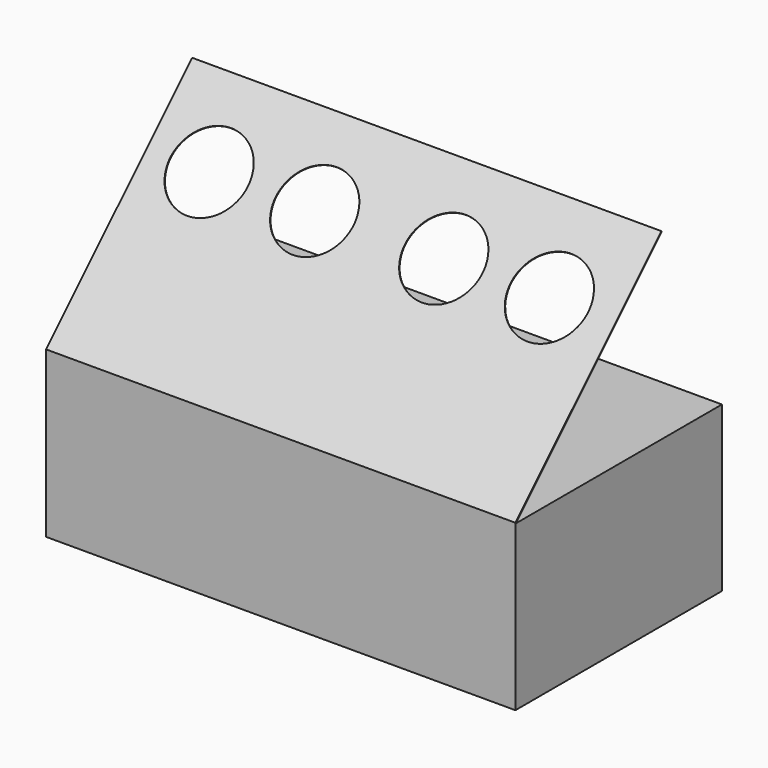
from build123d import *

# Parameters (mm, degrees)
F1_DEPTH = 127
F3_DEPTH = 0.4064


# Not quite as in the source:
# - the dataset's text gives a spline's control points without its knots; the knots are read off the source's solid


with BuildPart() as f1:
    # F0 (on Right) → F1 (new body, symmetric)
    with BuildSketch(Plane.YZ):
        Polygon((-139.7, 0), (0, 0), (0, 88.9), (-139.2936, 88.9), (-139.2936, 89.154), (-40.6298144724, 187.8177855276), (-40.9171826682, 188.1051537235), (-139.7, 89.3223363917), align=None)
    extrude(amount=F1_DEPTH, both=True)

    # F2 (on face) → F3 (cut, through all)
    with BuildSketch(Plane(origin=(0, -114.5111681959, 114.5111681959), x_dir=(1, 0, 0), z_dir=(0, -0.7071067812, 0.7071067812))):
        with BuildLine():
            add(Edge.make_bspline(
                [(-21.0882612312, 45.5766371575), (-17.1946190312, 49.4705841575), (-14.9277452312, 54.9434713575), (-14.9277452312, 60.4501405575), (-14.9277452312, 65.9570891575), (-17.1946190312, 71.4299763575), (-21.0882612312, 75.3236185575), (-24.9822590312, 79.2176163575), (-30.4551462312, 81.4845155575), (-35.9621202312, 81.4845155575)],
                knots=[5, 5, 5, 5, 6, 6, 6, 7, 7, 7, 8, 8, 8, 8], degree=3))
            add(Edge.make_bspline(
                [(-35.9621202312, 81.4845155575), (-41.4687640312, 81.4845155575), (-46.9416512312, 79.2176163575), (-50.8352934312, 75.3236185575)],
                knots=[0, 0, 0, 0, 1, 1, 1, 1], degree=3))
            add(Edge.make_bspline(
                [(-50.8352934312, 75.3236185575), (-54.7292912312, 71.4299763575), (-56.9964952312, 65.9570891575), (-56.9964952312, 60.4501405575), (-56.9964952312, 54.9434713575), (-54.7292912312, 49.4705841575), (-50.8352934312, 45.5766371575)],
                knots=[1, 1, 1, 1, 2, 2, 2, 3, 3, 3, 3], degree=3))
            add(Edge.make_bspline(
                [(-50.8352934312, 45.5766371575), (-46.9416512312, 41.6829441575), (-41.4687640312, 39.4157655575), (-35.9621202312, 39.4157655575), (-30.4551462312, 39.4157655575), (-24.9822590312, 41.6829441575), (-21.0882612312, 45.5766371575)],
                knots=[3, 3, 3, 3, 4, 4, 4, 5, 5, 5, 5], degree=3))
        make_face()
        with BuildLine():
            add(Edge.make_bspline(
                [(48.7617387688, 45.5766371575), (52.6553809688, 49.4705841575), (54.9222547688, 54.9434713575), (54.9222547688, 60.4501405575), (54.9222547688, 65.9570891575), (52.6553809688, 71.4299763575), (48.7617387688, 75.3236185575), (44.8677409688, 79.2176163575), (39.3948537688, 81.4845155575), (33.8878797688, 81.4845155575)],
                knots=[5, 5, 5, 5, 6, 6, 6, 7, 7, 7, 8, 8, 8, 8], degree=3))
            add(Edge.make_bspline(
                [(33.8878797688, 81.4845155575), (28.3812359688, 81.4845155575), (22.9083487688, 79.2176163575), (19.0147065688, 75.3236185575)],
                knots=[0, 0, 0, 0, 1, 1, 1, 1], degree=3))
            add(Edge.make_bspline(
                [(19.0147065688, 75.3236185575), (15.1207087688, 71.4299763575), (12.8535047688, 65.9570891575), (12.8535047688, 60.4501405575), (12.8535047688, 54.9434713575), (15.1207087688, 49.4705841575), (19.0147065688, 45.5766371575)],
                knots=[1, 1, 1, 1, 2, 2, 2, 3, 3, 3, 3], degree=3))
            add(Edge.make_bspline(
                [(19.0147065688, 45.5766371575), (22.9083487688, 41.6829441575), (28.3812359688, 39.4157655575), (33.8878797688, 39.4157655575), (39.3948537688, 39.4157655575), (44.8677409688, 41.6829441575), (48.7617387688, 45.5766371575)],
                knots=[3, 3, 3, 3, 4, 4, 4, 5, 5, 5, 5], degree=3))
        make_face()
        with BuildLine():
            add(Edge.make_bspline(
                [(105.9117387688, 45.5766371575), (109.8053809688, 49.4705841575), (112.0722547688, 54.9434713575), (112.0722547688, 60.4501405575), (112.0722547688, 65.9570891575), (109.8053809688, 71.4299763575), (105.9117387688, 75.3236185575), (102.0177409688, 79.2176163575), (96.5448537688, 81.4845155575), (91.0378797688, 81.4845155575)],
                knots=[5, 5, 5, 5, 6, 6, 6, 7, 7, 7, 8, 8, 8, 8], degree=3))
            add(Edge.make_bspline(
                [(91.0378797688, 81.4845155575), (85.5312359688, 81.4845155575), (80.0583487688, 79.2176163575), (76.1647065688, 75.3236185575)],
                knots=[0, 0, 0, 0, 1, 1, 1, 1], degree=3))
            add(Edge.make_bspline(
                [(76.1647065688, 75.3236185575), (72.2707087688, 71.4299763575), (70.0035047688, 65.9570891575), (70.0035047688, 60.4501405575), (70.0035047688, 54.9434713575), (72.2707087688, 49.4705841575), (76.1647065688, 45.5766371575)],
                knots=[1, 1, 1, 1, 2, 2, 2, 3, 3, 3, 3], degree=3))
            add(Edge.make_bspline(
                [(76.1647065688, 45.5766371575), (80.0583487688, 41.6829441575), (85.5312359688, 39.4157655575), (91.0378797688, 39.4157655575), (96.5448537688, 39.4157655575), (102.0177409688, 41.6829441575), (105.9117387688, 45.5766371575)],
                knots=[3, 3, 3, 3, 4, 4, 4, 5, 5, 5, 5], degree=3))
        make_face()
        with BuildLine():
            add(Edge.make_bspline(
                [(-78.2382612312, 45.5766371575), (-74.3446190312, 49.4705841575), (-72.0777452312, 54.9434713575), (-72.0777452312, 60.4501405575), (-72.0777452312, 65.9570891575), (-74.3446190312, 71.4299763575), (-78.2382612312, 75.3236185575), (-82.1322590312, 79.2176163575), (-87.6051462312, 81.4845155575), (-93.1121202312, 81.4845155575)],
                knots=[5, 5, 5, 5, 6, 6, 6, 7, 7, 7, 8, 8, 8, 8], degree=3))
            add(Edge.make_bspline(
                [(-93.1121202312, 81.4845155575), (-98.6187640312, 81.4845155575), (-104.0916512312, 79.2176163575), (-107.9855982312, 75.3236185575)],
                knots=[0, 0, 0, 0, 1, 1, 1, 1], degree=3))
            add(Edge.make_bspline(
                [(-107.9855982312, 75.3236185575), (-111.8792912312, 71.4299763575), (-114.1464952312, 65.9570891575), (-114.1464952312, 60.4501405575), (-114.1464952312, 54.9434713575), (-111.8792912312, 49.4705841575), (-107.9855982312, 45.5766371575)],
                knots=[1, 1, 1, 1, 2, 2, 2, 3, 3, 3, 3], degree=3))
            add(Edge.make_bspline(
                [(-107.9855982312, 45.5766371575), (-104.0916512312, 41.6829441575), (-98.6187640312, 39.4157655575), (-93.1121202312, 39.4157655575), (-87.6051462312, 39.4157655575), (-82.1322590312, 41.6829441575), (-78.2382612312, 45.5766371575)],
                knots=[3, 3, 3, 3, 4, 4, 4, 5, 5, 5, 5], degree=3))
        make_face()
    extrude(amount=-F3_DEPTH, mode=Mode.SUBTRACT)


solid = f1.part
